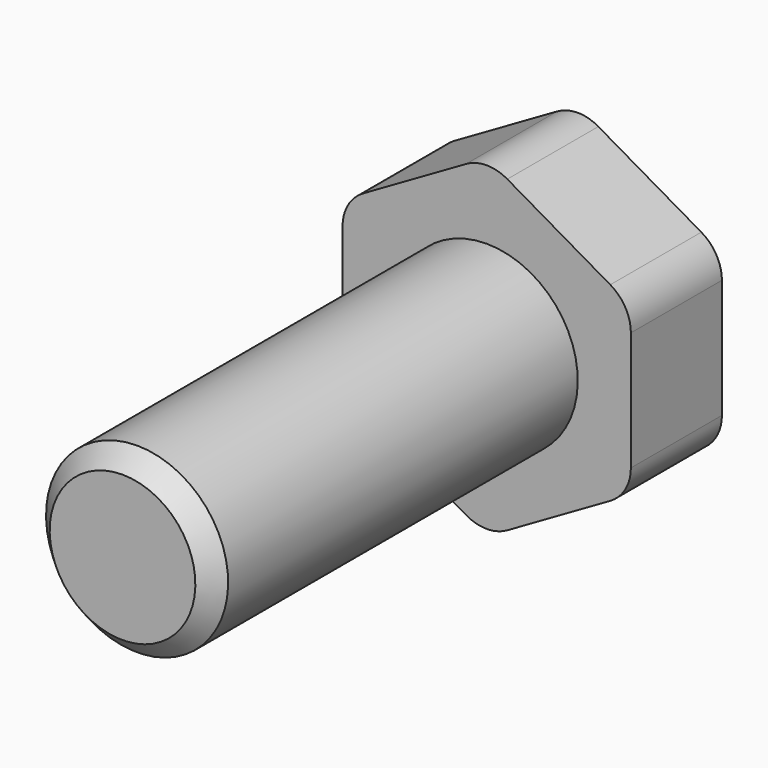
from build123d import *

# Parameters (mm, degrees)
F2_R     = 15.825
F3_DEPTH = 25


# Not quite as in the source:
# - a feature names something its author has since deleted; it is built from what else it names


with BuildPart() as f1:
    # F0 (on Right) → F1 (revolve)
    with BuildSketch(Plane.YZ):
        Polygon((0, 15.825), (0, 6), (-28.8, 6), (-30, 4.8), (-30, 0), (7.5, 0), (7.5, 15.825), align=None)
    revolve(axis=Axis((0, -11.25, 0), (0, -1, 0)))

    # F2 (on face) → F3 (cut)
    with BuildSketch(Plane(origin=(0, 7.5, 0), x_dir=(-1, 0, 0), z_dir=(0, 1, 0))):
        Circle(F2_R)
        with BuildLine():
            ThreePointArc((1.3563466521, -10.1865680099), (0, -10.55), (-1.3563466521, -10.1865680099))
            Line((-1.3563466521, -10.1865680099), (-8.1436533479, -6.267914662))
            ThreePointArc((-8.1436533479, -6.267914662), (-9.1365680099, -5.275), (-9.5, -3.9186533479))
            Line((-9.5, -3.9186533479), (-9.5, 3.9186533479))
            ThreePointArc((-9.5, 3.9186533479), (-9.1365680099, 5.275), (-8.1436533479, 6.267914662))
            Line((-8.1436533479, 6.267914662), (-1.3563466521, 10.1865680099))
            ThreePointArc((-1.3563466521, 10.1865680099), (0, 10.55), (1.3563466521, 10.1865680099))
            Line((1.3563466521, 10.1865680099), (8.1436533479, 6.267914662))
            ThreePointArc((8.1436533479, 6.267914662), (9.1365680099, 5.275), (9.5, 3.9186533479))
            Line((9.5, 3.9186533479), (9.5, -3.9186533479))
            ThreePointArc((9.5, -3.9186533479), (9.1365680099, -5.275), (8.1436533479, -6.267914662))
            Line((8.1436533479, -6.267914662), (1.3563466521, -10.1865680099))
        make_face(mode=Mode.SUBTRACT)
    extrude(amount=-F3_DEPTH, mode=Mode.SUBTRACT)


solid = f1.part
